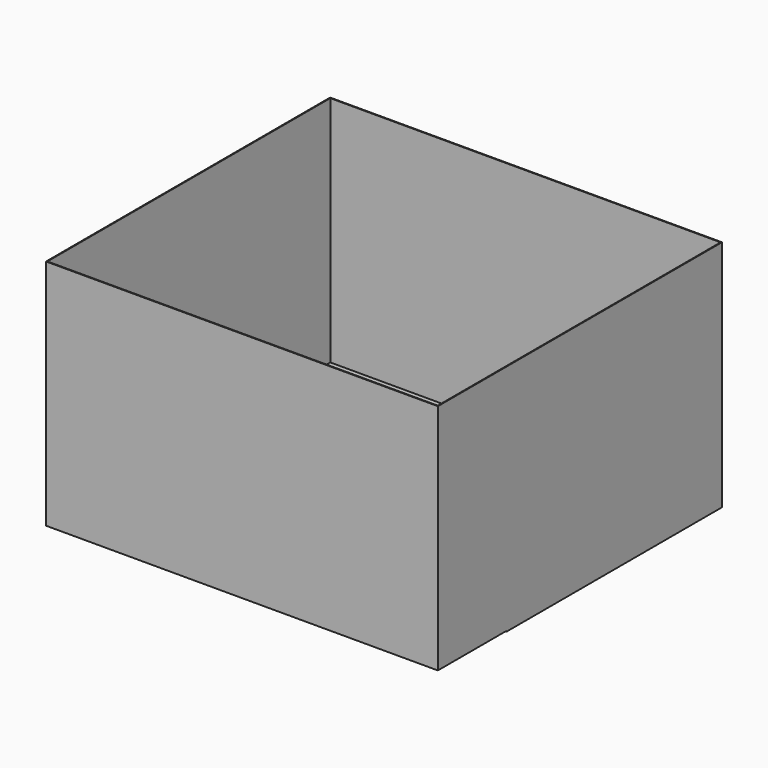
from build123d import *

# Parameters (mm, degrees)
F0_W     = 812.8
F0_H     = 482.6
F1_DEPTH = 1.524
F2_W     = 809.752
F2_H     = 1.524
F3_DEPTH = 482.6
F4_DEPTH = 254
F5_DEPTH = 254
F6_W     = 812.8
F6_H     = 177.8
F7_DEPTH = 1.524


with BuildPart() as f1:
    # F0 (on Top) → F1 (new body)
    with BuildSketch(Plane.XY):
        with Locations((-13.0345858634, -56.5100638679)):
            Rectangle(F0_W, F0_H)
    extrude(amount=F1_DEPTH)

    # F2 (on face) → F3 (join)
    with BuildSketch(Plane.XY.offset(1.524)):
        Polygon((393.3654141366, 184.7899361321), (391.8414141366, 184.7899361321), (391.8414141366, 183.2659361321), (391.8414141366, -296.2860638679), (391.8414141366, -297.8100638679), (393.3654141366, -297.8100638679), align=None)
        with Locations((-13.0345858634, 184.0279361321)):
            Rectangle(F2_W, F2_H)
        with Locations((-13.0345858634, -297.0480638679)):
            Rectangle(F2_W, F2_H)
        Polygon((-417.9105858634, 184.7899361321), (-419.4345858634, 184.7899361321), (-419.4345858634, -297.8100638679), (-417.9105858634, -297.8100638679), (-417.9105858634, -296.2860638679), (-417.9105858634, 183.2659361321), align=None)
    extrude(amount=F3_DEPTH)

    # F4 (add): a face of the model
    f4_faces = [f1.faces().sort_by_distance(p)[0] for p in [
        (-13.0345858634, -297.8100638679, 242.062),
    ]]
    extrude(f4_faces, amount=F4_DEPTH)

    # F5 (cut): a face of the model
    f5_faces = [f1.faces().sort_by_distance(p)[0] for p in [
        (-13.0345858634, -296.2860638679, 242.824),
    ]]
    extrude(f5_faces, amount=-F5_DEPTH, mode=Mode.SUBTRACT)

    # F6 (on face) → F7 (cut)
    with BuildSketch(Plane(origin=(0, 0, 0), x_dir=(1, 0, 0), z_dir=(0, 0, -1))):
        with Locations((-13.0345858634, 462.9100638679)):
            Rectangle(F6_W, F6_H)
    extrude(amount=-F7_DEPTH, mode=Mode.SUBTRACT)


solid = f1.part
